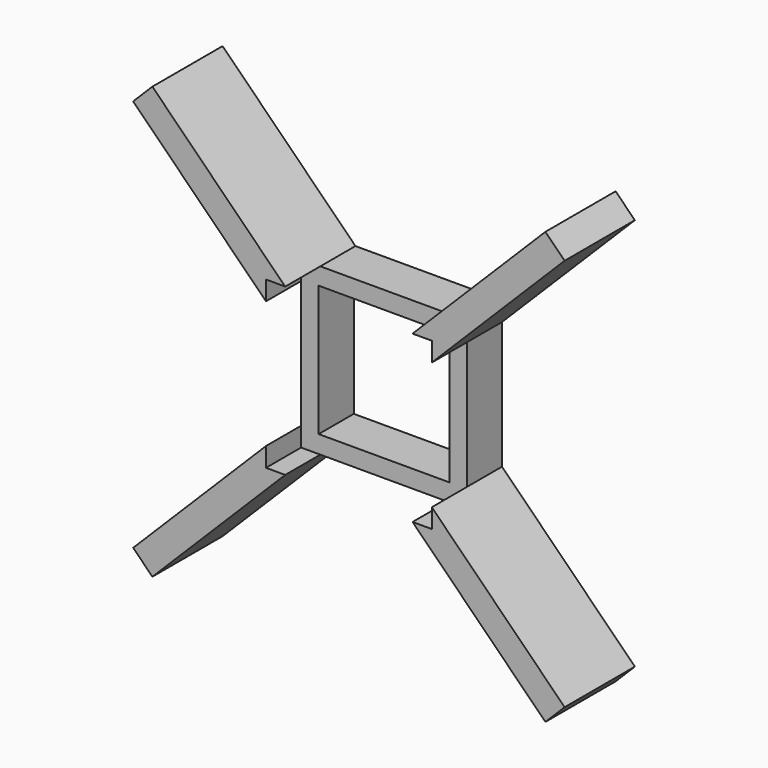
from build123d import *

# Parameters (mm, degrees)
F0_W     = 37.8080839926
F0_H     = 37.8080839926
F1_DEPTH = 12.7
F4_DEPTH = 25.4


# Not quite as in the source:
# - the program builds the solid bodies; features that only make, move or delete a surface that nothing else refers to are left out


with BuildPart() as f1:
    # F0 (on Front) → F1 (new body)
    with BuildSketch(Plane.XZ):
        Polygon((23.9840419963, 18.4223433702), (23.9840419963, 23.9840419963), (18.4223433702, 23.9840419963), (-18.4223433702, 23.9840419963), (-23.9840419963, 23.9840419963), (-23.9840419963, 18.4223433702), (-23.9840419963, -18.4223433702), (-23.9840419963, -23.9840419963), (-18.4223433702, -23.9840419963), (18.4223433702, -23.9840419963), (23.9840419963, -23.9840419963), (23.9840419963, -18.4223433702), align=None)
        Rectangle(F0_W, F0_H, mode=Mode.SUBTRACT)
    extrude(amount=F1_DEPTH)

    # F0 (on Front) → F4 (join)
    with BuildSketch(Plane.XZ):
        with BuildLine():
            Line((-23.9840419963, 23.9840419963), (-18.4223433702, 23.9840419963))
            Line((-18.4223433702, 23.9840419963), (-44.0913446559, 49.653043282))
            ThreePointArc((-44.0913446559, 49.653043282), (-46.5728804881, 46.5728804881), (-49.653043282, 44.0913446559))
            Line((-49.653043282, 44.0913446559), (-23.9840419963, 18.4223433702))
            Line((-23.9840419963, 18.4223433702), (-23.9840419963, 23.9840419963))
        make_face()
        with BuildLine():
            ThreePointArc((-49.653043282, 44.0913446559), (-46.5728804881, 46.5728804881), (-44.0913446559, 49.653043282))
            Line((-44.0913446559, 49.653043282), (-56.85978783, 62.4214864561))
            Line((-56.85978783, 62.4214864561), (-62.4214864561, 56.85978783))
            Line((-62.4214864561, 56.85978783), (-49.653043282, 44.0913446559))
        make_face()
        with BuildLine():
            ThreePointArc((-44.0913446559, -49.653043282), (-46.5728804881, -46.5728804881), (-49.653043282, -44.0913446559))
            Line((-49.653043282, -44.0913446559), (-62.4214864561, -56.85978783))
            Line((-62.4214864561, -56.85978783), (-56.85978783, -62.4214864561))
            Line((-56.85978783, -62.4214864561), (-44.0913446559, -49.653043282))
        make_face()
        with BuildLine():
            Line((-23.9840419963, -23.9840419963), (-23.9840419963, -18.4223433702))
            Line((-23.9840419963, -18.4223433702), (-49.653043282, -44.0913446559))
            ThreePointArc((-49.653043282, -44.0913446559), (-46.5728804881, -46.5728804881), (-44.0913446559, -49.653043282))
            Line((-44.0913446559, -49.653043282), (-18.4223433702, -23.9840419963))
            Line((-18.4223433702, -23.9840419963), (-23.9840419963, -23.9840419963))
        make_face()
        with BuildLine():
            Line((49.653043282, -44.0913446559), (23.9840419963, -18.4223433702))
            Line((23.9840419963, -18.4223433702), (23.9840419963, -23.9840419963))
            Line((23.9840419963, -23.9840419963), (18.4223433702, -23.9840419963))
            Line((18.4223433702, -23.9840419963), (44.0913446559, -49.653043282))
            ThreePointArc((44.0913446559, -49.653043282), (46.5728804881, -46.5728804881), (49.653043282, -44.0913446559))
        make_face()
        with BuildLine():
            Line((62.4214864561, -56.85978783), (49.653043282, -44.0913446559))
            ThreePointArc((49.653043282, -44.0913446559), (46.5728804881, -46.5728804881), (44.0913446559, -49.653043282))
            Line((44.0913446559, -49.653043282), (56.85978783, -62.4214864561))
            Line((56.85978783, -62.4214864561), (62.4214864561, -56.85978783))
        make_face()
        with BuildLine():
            Line((56.85978783, 62.4214864561), (44.0913446559, 49.653043282))
            ThreePointArc((44.0913446559, 49.653043282), (46.5728804881, 46.5728804881), (49.653043282, 44.0913446559))
            Line((49.653043282, 44.0913446559), (62.4214864561, 56.85978783))
            Line((62.4214864561, 56.85978783), (56.85978783, 62.4214864561))
        make_face()
        with BuildLine():
            Line((18.4223433702, 23.9840419963), (23.9840419963, 23.9840419963))
            Line((23.9840419963, 23.9840419963), (23.9840419963, 18.4223433702))
            Line((23.9840419963, 18.4223433702), (49.653043282, 44.0913446559))
            ThreePointArc((49.653043282, 44.0913446559), (46.5728804881, 46.5728804881), (44.0913446559, 49.653043282))
            Line((44.0913446559, 49.653043282), (18.4223433702, 23.9840419963))
        make_face()
    extrude(amount=F4_DEPTH)


solid = f1.part
